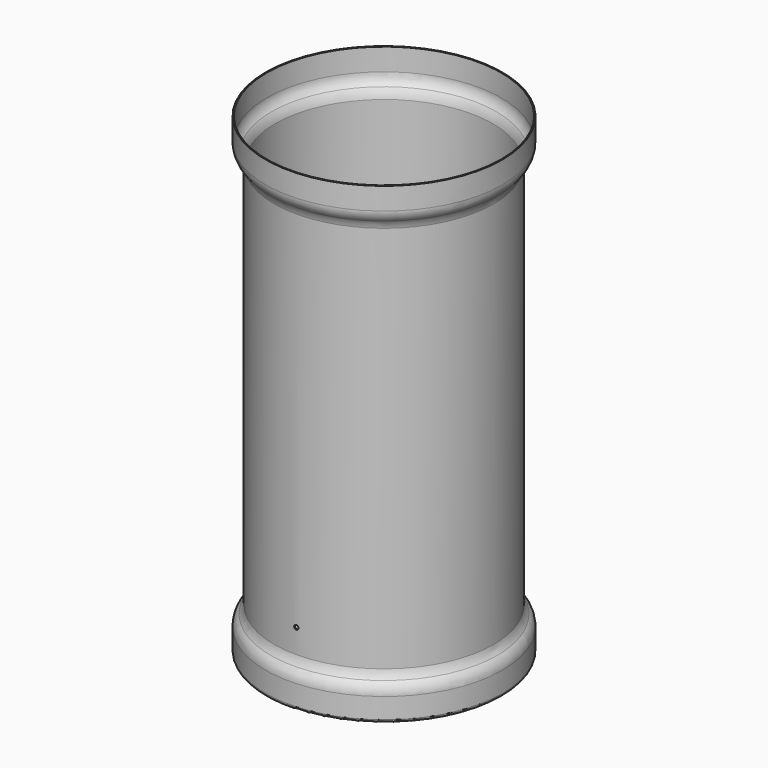
from build123d import *

# Parameters (mm, degrees)
F0_R     = 350
F1_DEPTH = 1400
F3_W     = 25.7771372795
F3_H     = 1181.948132813
F6_R     = 33.4608263206
F7_R     = 9.6568542495
F8_T     = -3
F2_R     = 6.35
F9_REACH = 367.9615123421


# Not quite as in the source:
# - a fillet or chamfer that OpenCascade refuses, or shapes differently, is made with other operations: its cross-section is extruded or revolved along the edge and cut away or added


with BuildPart() as f1:
    # F0 (on Top) → F1 (new body)
    with BuildSketch(Plane.XY):
        Circle(F0_R)
    extrude(amount=-F1_DEPTH)

    # F3 (on Front) → F4 (revolve, cut)
    with BuildSketch(Plane.XZ):
        with Locations((337.1114313602, -697.7157853544)):
            Rectangle(F3_W, F3_H)
    revolve(axis=Axis((0, 0, -700), (0, 0, -1)), mode=Mode.SUBTRACT)

    # F5: fillet of radius 45.8700576851 on 2 edges, made by hand

    # F5_s1 → F5_t2 (revolve, cut)
    with BuildSketch(Plane.XZ):
        with BuildLine():
            ThreePointArc((350, -65.5065793021), (343.0254793989, -89.8211713608), (324.2228627205, -106.7417189479))
            Line((324.2228627205, -106.7417189479), (350, -106.7417189479))
            Line((350, -106.7417189479), (350, -65.5065793021))
        make_face()
    revolve(axis=Axis((0, 0, -106.7417189479), (0, 0, -1)), mode=Mode.SUBTRACT)

    # F5_s3 → F5_t4 (revolve, cut)
    with BuildSketch(Plane.XZ):
        with BuildLine():
            ThreePointArc((324.2228627205, -1288.6898517609), (343.0254793989, -1305.6103993479), (350, -1329.9249914067))
            Line((350, -1329.9249914067), (350, -1288.6898517609))
            Line((350, -1288.6898517609), (324.2228627205, -1288.6898517609))
        make_face()
    revolve(axis=Axis((0, 0, -1288.6898517609), (0, 0, -1)), mode=Mode.SUBTRACT)

    # F6
    f6_edges = [f1.edges().sort_by_distance(p)[0] for p in [
        (-324.222863, 0, -106.741719),
        (324.222863, 0, -697.715785),
        (-324.222863, 0, -1288.689852),
    ]]
    fillet(f6_edges, radius=F6_R)

    # F7
    f7_edges = [f1.edges().sort_by_distance(p)[0] for p in [
        (-350, 0, -1400),
    ]]
    fillet(f7_edges, radius=F7_R)

    # F8
    f8_openings = [f1.faces().sort_by_distance(p)[0] for p in [
        (0, 0, 0),
    ]]
    offset(amount=F8_T, openings=f8_openings)

    f9_end = f1.faces().sort_by_distance((-324.2228627205, 0, -697.7157853554))[0]
    # F2 (on Front) → F9 (cut, up to a face of the model that its end follows)
    with BuildSketch(Plane.XZ):
        with Locations((0, -1200)):
            Circle(F2_R)
    f9_long = extrude(amount=F9_REACH, mode=Mode.PRIVATE)
    add(split(f9_long, bisect_by=f9_end, keep=Keep.BOTTOM, mode=Mode.PRIVATE), mode=Mode.SUBTRACT)


solid = f1.part
